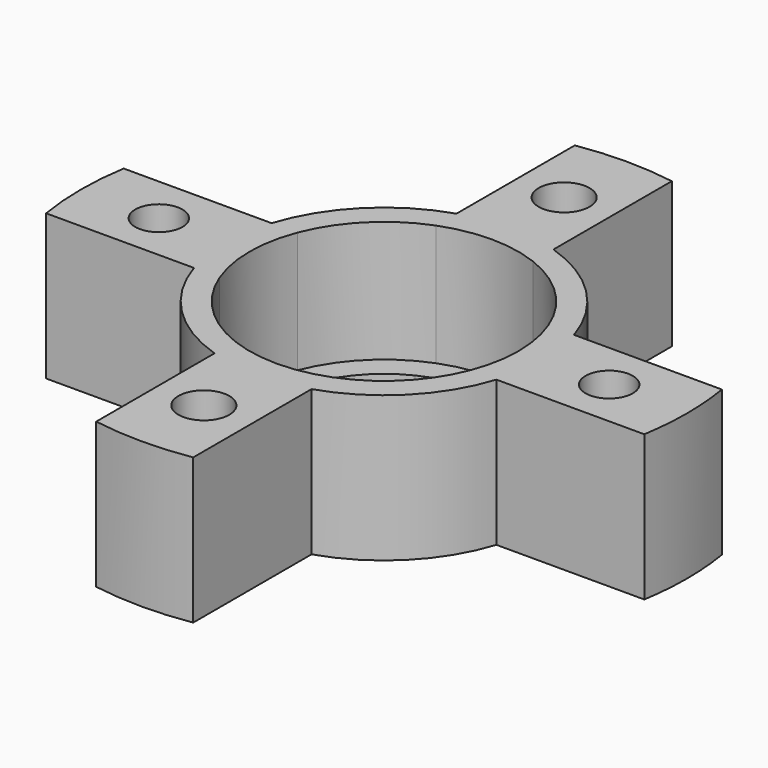
from build123d import *
from build123d import SkipClean  # not in build123d's __all__

# Parameters (mm, degrees)
F1_DEPTH = 2
F2_DEPTH = 10
F3_R     = 1.95
F3_R_2   = 2.1
F4_DEPTH = 12.001


# Not quite as in the source:
# - after a boolean that leaves OpenCascade's solid faulty, fix() repairs it


with BuildPart() as f1:
    # F0 (on Top) → F1 (new body)
    with BuildSketch(Plane.XY):
        with BuildLine():
            ThreePointArc((-4, 12.4743737318), (0, 13.1), (4, 12.4743737318))
            Line((4, 12.4743737318), (4, 24.6779253585))
            Line((4, 24.6779253585), (-4, 24.6779253585))
            Line((-4, 24.6779253585), (-4, 12.4743737318))
        make_face()
        with BuildLine():
            Line((-4, 24.6779253585), (4, 24.6779253585))
            ThreePointArc((4, 24.6779253585), (0, 25), (-4, 24.6779253585))
        make_face()
        with BuildLine():
            ThreePointArc((25, 0), (24.9193512552, 2.0064727804), (24.6779253585, 4))
            Line((24.6779253585, 4), (24.6779253585, -4))
            ThreePointArc((24.6779253585, -4), (24.9193512552, -2.0064727804), (25, 0))
        make_face()
        with BuildLine():
            Line((24.6779253585, 4), (12.4743737318, 4))
            ThreePointArc((12.4743737318, 4), (12.942648413, 2.0243152069), (13.1, 0))
            ThreePointArc((13.1, 0), (12.942648413, -2.0243152069), (12.4743737318, -4))
            Line((12.4743737318, -4), (24.6779253585, -4))
            Line((24.6779253585, -4), (24.6779253585, 4))
        make_face()
        with BuildLine():
            ThreePointArc((-4, -24.6779253585), (0, -25), (4, -24.6779253585))
            Line((4, -24.6779253585), (-4, -24.6779253585))
        make_face()
        with BuildLine():
            Line((-24.6779253585, -4), (-24.6779253585, 4))
            ThreePointArc((-24.6779253585, 4), (-25, 0), (-24.6779253585, -4))
        make_face()
        with BuildLine():
            ThreePointArc((-12.4743737318, -4), (-13.1, 0), (-12.4743737318, 4))
            Line((-12.4743737318, 4), (-24.6779253585, 4))
            Line((-24.6779253585, 4), (-24.6779253585, -4))
            Line((-24.6779253585, -4), (-12.4743737318, -4))
        make_face()
        with BuildLine():
            Line((4, -24.6779253585), (4, -12.4743737318))
            ThreePointArc((4, -12.4743737318), (0, -13.1), (-4, -12.4743737318))
            Line((-4, -12.4743737318), (-4, -24.6779253585))
            Line((-4, -24.6779253585), (4, -24.6779253585))
        make_face()
        with BuildLine():
            Line((-4, -12.4743737318), (-4, -10.3542261903))
            ThreePointArc((-4, -10.3542261903), (-7.8488852712, -7.8488852712), (-10.3542261903, -4))
            Line((-10.3542261903, -4), (-12.4743737318, -4))
            ThreePointArc((-12.4743737318, -4), (-9.2630988335, -9.2630988335), (-4, -12.4743737318))
        make_face()
        with BuildLine():
            ThreePointArc((-10.3542261903, -4), (-7.8488852712, -7.8488852712), (-4, -10.3542261903))
            Line((-4, -10.3542261903), (-4, -8.1737384348))
            ThreePointArc((-4, -8.1737384348), (-6.4346717088, -6.4346717088), (-8.1737384348, -4))
            Line((-8.1737384348, -4), (-10.3542261903, -4))
        make_face()
        with BuildLine():
            Line((-8.1737384348, 4), (-10.3542261903, 4))
            ThreePointArc((-10.3542261903, 4), (-11.1, 0), (-10.3542261903, -4))
            Line((-10.3542261903, -4), (-8.1737384348, -4))
            ThreePointArc((-8.1737384348, -4), (-9.1, 0), (-8.1737384348, 4))
        make_face()
        with BuildLine():
            ThreePointArc((-10.3542261903, -4), (-11.1, 0), (-10.3542261903, 4))
            Line((-10.3542261903, 4), (-12.4743737318, 4))
            ThreePointArc((-12.4743737318, 4), (-13.1, 0), (-12.4743737318, -4))
            Line((-12.4743737318, -4), (-10.3542261903, -4))
        make_face()
        with BuildLine():
            ThreePointArc((-10.3542261903, 4), (-7.8488852712, 7.8488852712), (-4, 10.3542261903))
            Line((-4, 10.3542261903), (-4, 12.4743737318))
            ThreePointArc((-4, 12.4743737318), (-9.2630988335, 9.2630988335), (-12.4743737318, 4))
            Line((-12.4743737318, 4), (-10.3542261903, 4))
        make_face()
        with BuildLine():
            Line((-4, 8.1737384348), (-4, 10.3542261903))
            ThreePointArc((-4, 10.3542261903), (-7.8488852712, 7.8488852712), (-10.3542261903, 4))
            Line((-10.3542261903, 4), (-8.1737384348, 4))
            ThreePointArc((-8.1737384348, 4), (-6.4346717088, 6.4346717088), (-4, 8.1737384348))
        make_face()
        with BuildLine():
            Line((4, 8.1737384348), (4, 10.3542261903))
            ThreePointArc((4, 10.3542261903), (0, 11.1), (-4, 10.3542261903))
            Line((-4, 10.3542261903), (-4, 8.1737384348))
            ThreePointArc((-4, 8.1737384348), (0, 9.1), (4, 8.1737384348))
        make_face()
        with BuildLine():
            ThreePointArc((-4, 10.3542261903), (0, 11.1), (4, 10.3542261903))
            Line((4, 10.3542261903), (4, 12.4743737318))
            ThreePointArc((4, 12.4743737318), (0, 13.1), (-4, 12.4743737318))
            Line((-4, 12.4743737318), (-4, 10.3542261903))
        make_face()
        with BuildLine():
            ThreePointArc((4, 10.3542261903), (7.8488852712, 7.8488852712), (10.3542261903, 4))
            Line((10.3542261903, 4), (12.4743737318, 4))
            ThreePointArc((12.4743737318, 4), (9.2630988335, 9.2630988335), (4, 12.4743737318))
            Line((4, 12.4743737318), (4, 10.3542261903))
        make_face()
        with BuildLine():
            Line((8.1737384348, 4), (10.3542261903, 4))
            ThreePointArc((10.3542261903, 4), (7.8488852712, 7.8488852712), (4, 10.3542261903))
            Line((4, 10.3542261903), (4, 8.1737384348))
            ThreePointArc((4, 8.1737384348), (6.4346717088, 6.4346717088), (8.1737384348, 4))
        make_face()
        with BuildLine():
            ThreePointArc((10.3542261903, 4), (10.9119638634, 2.0344642154), (11.1, 0))
            ThreePointArc((11.1, 0), (10.9119638634, -2.0344642154), (10.3542261903, -4))
            Line((10.3542261903, -4), (12.4743737318, -4))
            ThreePointArc((12.4743737318, -4), (12.942648413, -2.0243152069), (13.1, 0))
            ThreePointArc((13.1, 0), (12.942648413, 2.0243152069), (12.4743737318, 4))
            Line((12.4743737318, 4), (10.3542261903, 4))
        make_face()
        with BuildLine():
            ThreePointArc((10.3542261903, -4), (10.9119638634, -2.0344642154), (11.1, 0))
            ThreePointArc((11.1, 0), (10.9119638634, 2.0344642154), (10.3542261903, 4))
            Line((10.3542261903, 4), (8.1737384348, 4))
            ThreePointArc((8.1737384348, 4), (8.8654108691, 2.052922337), (9.1, 0))
            ThreePointArc((9.1, 0), (8.8654108691, -2.052922337), (8.1737384348, -4))
            Line((8.1737384348, -4), (10.3542261903, -4))
        make_face()
        with BuildLine():
            Line((12.4743737318, -4), (10.3542261903, -4))
            ThreePointArc((10.3542261903, -4), (7.8488852712, -7.8488852712), (4, -10.3542261903))
            Line((4, -10.3542261903), (4, -12.4743737318))
            ThreePointArc((4, -12.4743737318), (9.2630988335, -9.2630988335), (12.4743737318, -4))
        make_face()
        with BuildLine():
            ThreePointArc((4, -10.3542261903), (7.8488852712, -7.8488852712), (10.3542261903, -4))
            Line((10.3542261903, -4), (8.1737384348, -4))
            ThreePointArc((8.1737384348, -4), (6.4346717088, -6.4346717088), (4, -8.1737384348))
            Line((4, -8.1737384348), (4, -10.3542261903))
        make_face()
        with BuildLine():
            ThreePointArc((-4, -10.3542261903), (0, -11.1), (4, -10.3542261903))
            Line((4, -10.3542261903), (4, -8.1737384348))
            ThreePointArc((4, -8.1737384348), (0, -9.1), (-4, -8.1737384348))
            Line((-4, -8.1737384348), (-4, -10.3542261903))
        make_face()
        with BuildLine():
            Line((4, -12.4743737318), (4, -10.3542261903))
            ThreePointArc((4, -10.3542261903), (0, -11.1), (-4, -10.3542261903))
            Line((-4, -10.3542261903), (-4, -12.4743737318))
            ThreePointArc((-4, -12.4743737318), (0, -13.1), (4, -12.4743737318))
        make_face()
    extrude(amount=-F1_DEPTH)

    # F0 (on Top) → F2 (join)
    with BuildSketch(Plane.XY):
        with BuildLine():
            ThreePointArc((-4, 10.3542261903), (0, 11.1), (4, 10.3542261903))
            Line((4, 10.3542261903), (4, 12.4743737318))
            ThreePointArc((4, 12.4743737318), (0, 13.1), (-4, 12.4743737318))
            Line((-4, 12.4743737318), (-4, 10.3542261903))
        make_face()
        with BuildLine():
            ThreePointArc((4, 10.3542261903), (7.8488852712, 7.8488852712), (10.3542261903, 4))
            Line((10.3542261903, 4), (12.4743737318, 4))
            ThreePointArc((12.4743737318, 4), (9.2630988335, 9.2630988335), (4, 12.4743737318))
            Line((4, 12.4743737318), (4, 10.3542261903))
        make_face()
        with BuildLine():
            ThreePointArc((-4, 12.4743737318), (0, 13.1), (4, 12.4743737318))
            Line((4, 12.4743737318), (4, 24.6779253585))
            Line((4, 24.6779253585), (-4, 24.6779253585))
            Line((-4, 24.6779253585), (-4, 12.4743737318))
        make_face()
        with BuildLine():
            ThreePointArc((-10.3542261903, 4), (-7.8488852712, 7.8488852712), (-4, 10.3542261903))
            Line((-4, 10.3542261903), (-4, 12.4743737318))
            ThreePointArc((-4, 12.4743737318), (-9.2630988335, 9.2630988335), (-12.4743737318, 4))
            Line((-12.4743737318, 4), (-10.3542261903, 4))
        make_face()
        with BuildLine():
            ThreePointArc((-10.3542261903, -4), (-11.1, 0), (-10.3542261903, 4))
            Line((-10.3542261903, 4), (-12.4743737318, 4))
            ThreePointArc((-12.4743737318, 4), (-13.1, 0), (-12.4743737318, -4))
            Line((-12.4743737318, -4), (-10.3542261903, -4))
        make_face()
        with BuildLine():
            ThreePointArc((-12.4743737318, -4), (-13.1, 0), (-12.4743737318, 4))
            Line((-12.4743737318, 4), (-24.6779253585, 4))
            Line((-24.6779253585, 4), (-24.6779253585, -4))
            Line((-24.6779253585, -4), (-12.4743737318, -4))
        make_face()
        with BuildLine():
            Line((-4, -12.4743737318), (-4, -10.3542261903))
            ThreePointArc((-4, -10.3542261903), (-7.8488852712, -7.8488852712), (-10.3542261903, -4))
            Line((-10.3542261903, -4), (-12.4743737318, -4))
            ThreePointArc((-12.4743737318, -4), (-9.2630988335, -9.2630988335), (-4, -12.4743737318))
        make_face()
        with BuildLine():
            Line((4, -12.4743737318), (4, -10.3542261903))
            ThreePointArc((4, -10.3542261903), (0, -11.1), (-4, -10.3542261903))
            Line((-4, -10.3542261903), (-4, -12.4743737318))
            ThreePointArc((-4, -12.4743737318), (0, -13.1), (4, -12.4743737318))
        make_face()
        with BuildLine():
            Line((4, -24.6779253585), (4, -12.4743737318))
            ThreePointArc((4, -12.4743737318), (0, -13.1), (-4, -12.4743737318))
            Line((-4, -12.4743737318), (-4, -24.6779253585))
            Line((-4, -24.6779253585), (4, -24.6779253585))
        make_face()
        with BuildLine():
            Line((12.4743737318, -4), (10.3542261903, -4))
            ThreePointArc((10.3542261903, -4), (7.8488852712, -7.8488852712), (4, -10.3542261903))
            Line((4, -10.3542261903), (4, -12.4743737318))
            ThreePointArc((4, -12.4743737318), (9.2630988335, -9.2630988335), (12.4743737318, -4))
        make_face()
        with BuildLine():
            ThreePointArc((10.3542261903, 4), (10.9119638634, 2.0344642154), (11.1, 0))
            ThreePointArc((11.1, 0), (10.9119638634, -2.0344642154), (10.3542261903, -4))
            Line((10.3542261903, -4), (12.4743737318, -4))
            ThreePointArc((12.4743737318, -4), (12.942648413, -2.0243152069), (13.1, 0))
            ThreePointArc((13.1, 0), (12.942648413, 2.0243152069), (12.4743737318, 4))
            Line((12.4743737318, 4), (10.3542261903, 4))
        make_face()
        with BuildLine():
            Line((24.6779253585, 4), (12.4743737318, 4))
            ThreePointArc((12.4743737318, 4), (12.942648413, 2.0243152069), (13.1, 0))
            ThreePointArc((13.1, 0), (12.942648413, -2.0243152069), (12.4743737318, -4))
            Line((12.4743737318, -4), (24.6779253585, -4))
            Line((24.6779253585, -4), (24.6779253585, 4))
        make_face()
        with BuildLine():
            ThreePointArc((25, 0), (24.9193512552, 2.0064727804), (24.6779253585, 4))
            Line((24.6779253585, 4), (24.6779253585, -4))
            ThreePointArc((24.6779253585, -4), (24.9193512552, -2.0064727804), (25, 0))
        make_face()
        with BuildLine():
            ThreePointArc((-4, -24.6779253585), (0, -25), (4, -24.6779253585))
            Line((4, -24.6779253585), (-4, -24.6779253585))
        make_face()
        with BuildLine():
            Line((-24.6779253585, -4), (-24.6779253585, 4))
            ThreePointArc((-24.6779253585, 4), (-25, 0), (-24.6779253585, -4))
        make_face()
        with BuildLine():
            Line((-4, 24.6779253585), (4, 24.6779253585))
            ThreePointArc((4, 24.6779253585), (0, 25), (-4, 24.6779253585))
        make_face()
    with SkipClean():  # cleaning this boolean's faces spoils the solid; the shape is the same uncleaned
        extrude(amount=F2_DEPTH)

    # F3 (on face) → F4 (cut, through all)
    with BuildSketch(Plane.XY.offset(10)):
        with Locations((18.5761495451, 0)):
            Circle(F3_R)
        with Locations((0, 18.5761495451)):
            Circle(F3_R_2)
        with Locations((0, -18.5761495451)):
            Circle(F3_R_2)
        with Locations((-18.5761495451, 0)):
            Circle(F3_R)
    extrude(amount=-F4_DEPTH, mode=Mode.SUBTRACT)

    add(f1.part.fix(), mode=Mode.REPLACE)


solid = f1.part
